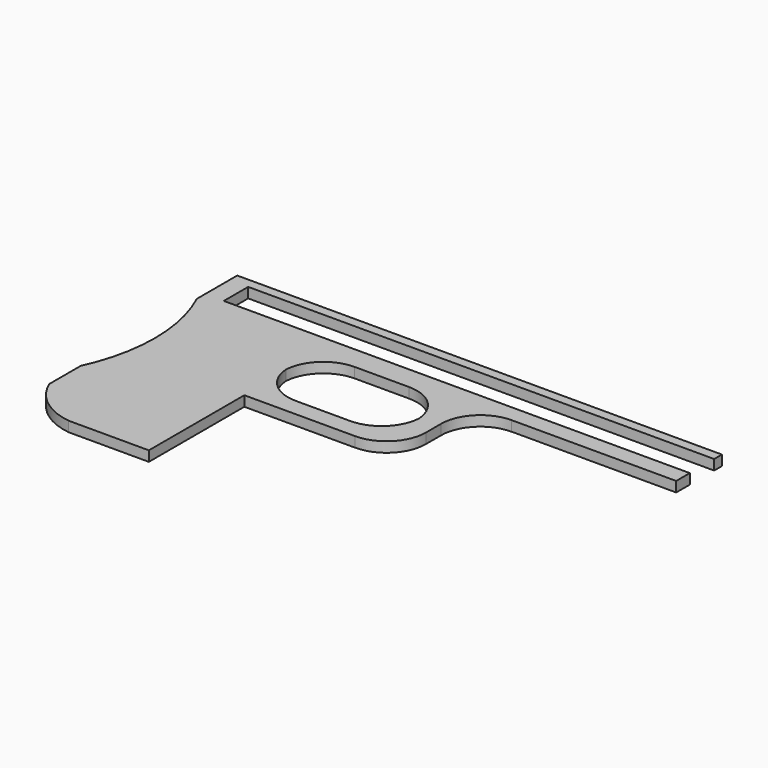
from build123d import *

# Parameters (mm, degrees)
F0_W         = 142.9656147957
F0_H         = 80.8112323284
F1_DEPTH     = 3
F2_W         = 137.4550536275
F2_H         = 8.9848991483
F2_W_2       = 60.0944850594
F2_H_2       = 18.4983238578
F3_DEPTH     = 52.3
F4_W         = 39.2408655025
F4_H         = 21.6958951205
F5_DEPTH     = 25
F6_W         = 3.3521875739
F6_H         = 44.7733802721
F6_W_2       = 40.9712046385
F7_DEPTH     = 25
F8_W         = 102.604271844
F8_H         = 18.422623165
F9_DEPTH     = 25
F10_T1_DEPTH = 3
F10_T3_DEPTH = 60.941125497
F12_DEPTH    = 25
F14_DEPTH    = 25
F16_DEPTH    = 25


# Not quite as in the source:
# - a fillet or chamfer that OpenCascade refuses, or shapes differently, is made with other operations: its cross-section is extruded or revolved along the edge and cut away or added


with BuildPart() as f1:
    # F0 (on Top) → F1 (new body)
    with BuildSketch(Plane.XY):
        Rectangle(F0_W, F0_H)
    extrude(amount=F1_DEPTH)

    # F2 (on face) → F3 (cut)
    with BuildSketch(Plane.XY.offset(3)):
        with Locations((2.7552805841, 33.0591509119)):
            Rectangle(F2_W, F2_H)
        with Locations((41.4355648682, 14.2965670675)):
            Rectangle(F2_W_2, F2_H_2)
    extrude(amount=-F3_DEPTH, mode=Mode.SUBTRACT)

    # F4 (on face) → F5 (cut)
    with BuildSketch(Plane.XY.offset(3)):
        with Locations((-13.8379565906, 10.8479475603)):
            Rectangle(F4_W, F4_H)
    extrude(amount=-F5_DEPTH, mode=Mode.SUBTRACT)

    # F6 (on face) → F7 (cut)
    with BuildSketch(Plane.XY.offset(3)):
        Polygon((98.6725464463, 0), (13.7504395097, 0), (13.7504395097, -5.2010240033), (17.1026270837, -5.2010240033), (17.1026270837, -49.9744042754), (13.7504395097, -49.9744042754), (13.7504395097, -55.2418604493), (98.6725464463, -55.2418604493), align=None)
        with Locations((15.4265332967, -27.5877141394)):
            Rectangle(F6_W, F6_H)
        with Locations((-6.7351628095, -27.5877141394)):
            Rectangle(F6_W_2, F6_H)
    extrude(amount=-F7_DEPTH, mode=Mode.SUBTRACT)

    # F8 (on face) → F9 (cut)
    with BuildSketch(Plane.XY.offset(3)):
        with Locations((62.6904582605, -4.1639064439)):
            Rectangle(F8_W, F8_H)
    extrude(amount=-F9_DEPTH, mode=Mode.SUBTRACT)

    # F10: fillet of radius 11.5882250994 on 7 edges, made by hand

    # F10_s2 → F10_t1 (join)
    with BuildSketch(Plane.XY):
        with BuildLine():
            ThreePointArc((22.9765474379, 23.5457289964), (14.7824348882, 20.1516164467), (11.3883223385, 11.957503897))
            Line((11.3883223385, 11.957503897), (11.3883223385, 23.5457289964))
            Line((11.3883223385, 23.5457289964), (22.9765474379, 23.5457289964))
        make_face()
        with BuildLine():
            ThreePointArc((-15.6325400293, -5.2010240033), (-23.826652579, -8.595136553), (-27.2207651287, -16.7892491027))
            Line((-27.2207651287, -16.7892491027), (-27.2207651287, -5.2010240033))
            Line((-27.2207651287, -5.2010240033), (-15.6325400293, -5.2010240033))
        make_face()
        with BuildLine():
            ThreePointArc((-33.4583893418, 10.1076700211), (-30.0642767921, 18.3017825708), (-21.8701642424, 21.6958951205))
            Line((-21.8701642424, 21.6958951205), (-33.4583893418, 21.6958951205))
            Line((-33.4583893418, 21.6958951205), (-33.4583893418, 10.1076700211))
        make_face()
        with BuildLine():
            ThreePointArc((-5.8057489387, 0), (2.388363611, 3.3941125497), (5.7824761607, 11.5882250994))
            Line((5.7824761607, 11.5882250994), (5.7824761607, 0))
            Line((5.7824761607, 0), (-5.8057489387, 0))
        make_face()
        with BuildLine():
            ThreePointArc((-33.4583893418, 11.5882250994), (-30.0642767921, 3.3941125497), (-21.8701642424, 0))
            Line((-21.8701642424, 0), (-33.4583893418, 0))
            Line((-33.4583893418, 0), (-33.4583893418, 11.5882250994))
        make_face()
        with BuildLine():
            ThreePointArc((5.7824761607, 10.1076700211), (2.388363611, 18.3017825708), (-5.8057489387, 21.6958951205))
            Line((-5.8057489387, 21.6958951205), (5.7824761607, 21.6958951205))
            Line((5.7824761607, 21.6958951205), (5.7824761607, 10.1076700211))
        make_face()
    extrude(amount=F10_T1_DEPTH)

    # F10_s4 → F10_t3 (cut)
    with BuildSketch(Plane.XY.offset(-28.9705627485)):
        with BuildLine():
            ThreePointArc((-0.1999027609, -5.2010240033), (7.9942097888, -1.8069114536), (11.3883223385, 6.3872010961))
            Line((11.3883223385, 6.3872010961), (11.3883223385, -5.2010240033))
            Line((11.3883223385, -5.2010240033), (-0.1999027609, -5.2010240033))
        make_face()
    extrude(amount=F10_T3_DEPTH, mode=Mode.SUBTRACT)

    # F11 (on face) → F12 (cut)
    with BuildSketch(Plane.XY.offset(3)):
        with BuildLine():
            Line((-71.4828073978, 25.5012605339), (-71.4828073978, -17.3091441393))
            ThreePointArc((-71.4828073978, -17.3091441393), (-66.7668008007, 4.0960581973), (-71.4828073978, 25.5012605339))
        make_face()
    extrude(amount=-F12_DEPTH, mode=Mode.SUBTRACT)

    # F13 (on face) → F14 (cut)
    with BuildSketch(Plane.XY.offset(3)):
        with BuildLine():
            ThreePointArc((-21.3245461018, -6.6952891353), (-30.1185964093, -13.4662376926), (-27.2207651287, -24.1799503565))
            Line((-27.2207651287, -24.1799503565), (-27.2207651287, -16.7892491027))
            ThreePointArc((-27.2207651287, -16.7892491027), (-25.6387183355, -10.944306275), (-21.3245461018, -6.6952891353))
        make_face()
        with BuildLine():
            ThreePointArc((-27.2207651287, -32.8327932205), (-29.4171017882, -37.101902666), (-32.9005867243, -40.4056161642))
            Line((-32.9005867243, -40.4056161642), (-27.2207651287, -40.4056161642))
            Line((-27.2207651287, -40.4056161642), (-27.2207651287, -32.8327932205))
        make_face()
        with BuildLine():
            ThreePointArc((-56.574376872, -40.4056161642), (-65.5880780241, -36.6447482344), (-71.4828073978, -28.8573801517))
            Line((-71.4828073978, -28.8573801517), (-71.4828073978, -40.4056161642))
            Line((-71.4828073978, -40.4056161642), (-56.574376872, -40.4056161642))
        make_face()
    extrude(amount=-F14_DEPTH, mode=Mode.SUBTRACT)

    # F15 (on face) → F16 (cut)
    with BuildSketch(Plane.XY.offset(3)):
        with BuildLine():
            Line((-32.9005867243, -5.2010240033), (-32.9005867243, -40.4056161642))
            ThreePointArc((-32.9005867243, -40.4056161642), (-29.4171017882, -37.101902666), (-27.2207651287, -32.8327932205))
            Line((-27.2207651287, -32.8327932205), (-27.2207651287, -24.1799503565))
            ThreePointArc((-27.2207651287, -24.1799503565), (-30.1185964093, -13.4662376926), (-21.3245461018, -6.6952891353))
            ThreePointArc((-21.3245461018, -6.6952891353), (-18.5749778542, -5.5808138595), (-15.6325400293, -5.2010240033))
            Line((-15.6325400293, -5.2010240033), (-32.9005867243, -5.2010240033))
        make_face()
    extrude(amount=-F16_DEPTH, mode=Mode.SUBTRACT)


solid = f1.part
